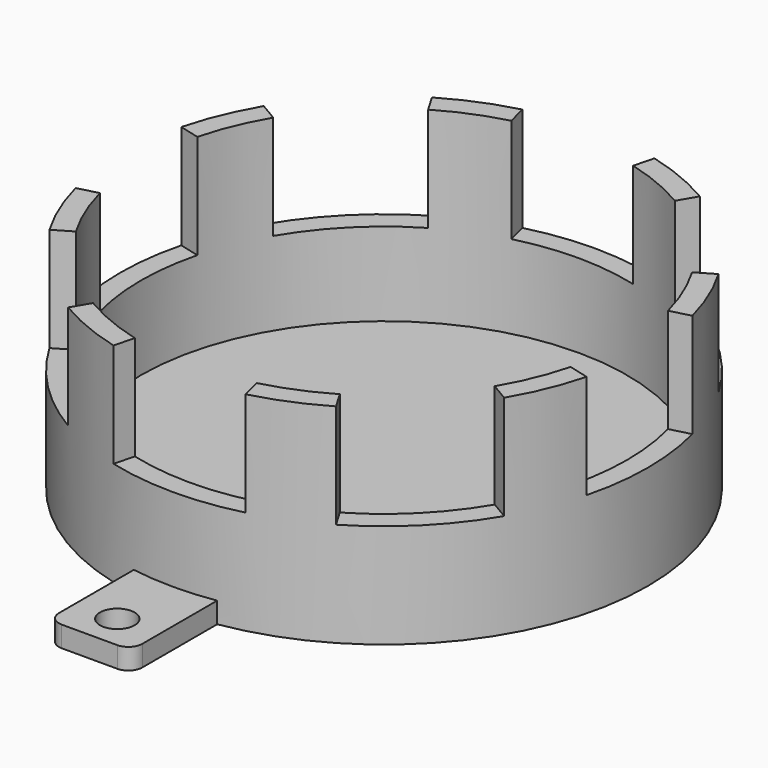
from build123d import *

# Parameters (mm, degrees)
F0_R            = 38
F1_DEPTH        = 3
F2_R            = 38
F2_R_2          = 35
F3_DEPTH        = 27
F4_W            = 12
F4_H            = 23
F4_R            = 2.5
F5_DEPTH        = 3
F6_R            = 2
F8_DEPTH        = 15
F8_COPIES_COUNT = 8


# Not quite as in the source:
# - a pattern or mirror of a feature is missing from the dataset's text; its kind, count and spacing are read off the source's solid


with BuildPart() as f1:
    # F0 (on Top) → F1 (new body)
    with BuildSketch(Plane.XY):
        Circle(F0_R)
    extrude(amount=F1_DEPTH)

    # F2 (on face) → F3 (join)
    with BuildSketch(Plane.XY.offset(3)):
        Circle(F2_R)
        Circle(F2_R_2, mode=Mode.SUBTRACT)
    extrude(amount=F3_DEPTH)

    # F4 (on Top) → F5 (join)
    with BuildSketch(Plane.XY):
        with Locations((0, -41.5)):
            Rectangle(F4_W, F4_H)
        with Locations((0, -48)):
            Circle(F4_R, mode=Mode.SUBTRACT)
    extrude(amount=F5_DEPTH)

    # F6
    f6_edges = [f1.edges().sort_by_distance(p)[0] for p in [
        (6, -53, 1.5),
        (-6, -53, 1.5),
    ]]
    fillet(f6_edges, radius=F6_R)

    # F7 (on face) → F8 (cut)
    with BuildSketch(Plane.XY.offset(30)):
        with BuildLine():
            Line((-9.5144401541, 36.7896103344), (-8.7633001419, 33.8851674132))
            ThreePointArc((-8.7633001419, 33.8851674132), (0, 35), (8.7633001419, 33.8851674132))
            Line((8.7633001419, 33.8851674132), (9.5144401541, 36.7896103344))
            ThreePointArc((9.5144401541, 36.7896103344), (0, 38), (-9.5144401541, 36.7896103344))
        make_face()
    f8 = extrude(amount=-F8_DEPTH, mode=Mode.SUBTRACT)

    # F8_copies: F8 ×8 about axis
    f8_copies_axis = Axis((0, 0, 0), (0, 0, 1))
    for i in range(1, F8_COPIES_COUNT):
        add(f8.rotate(f8_copies_axis, i * 360 / F8_COPIES_COUNT), mode=Mode.SUBTRACT)


solid = f1.part
